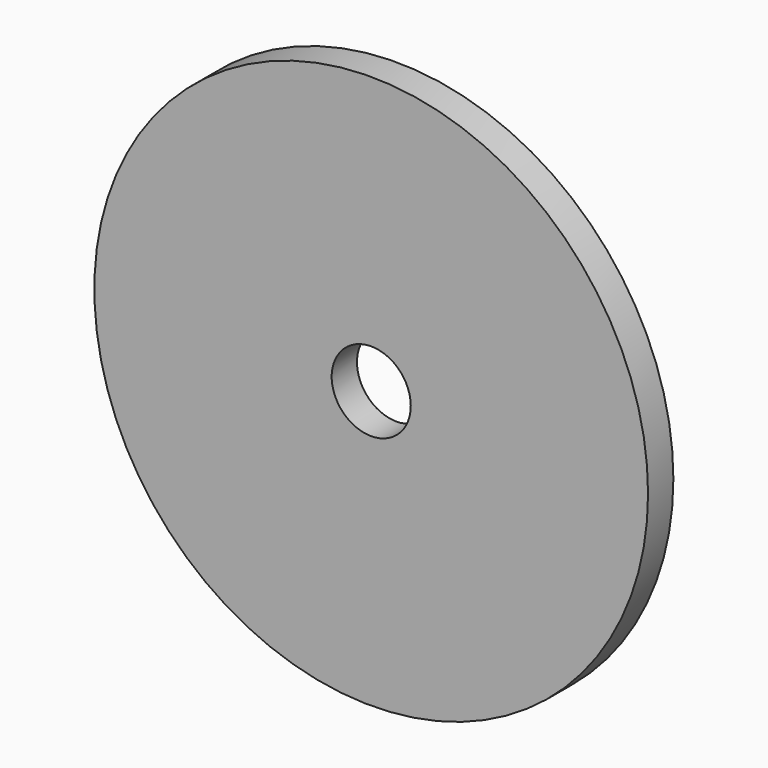
from build123d import *

# Parameters (mm, degrees)
F0_R     = 17.5
F1_DEPTH = 2.00000108
F2_R     = 2.5
F3_DEPTH = 6
F6_DEPTH = 8.00100108


# Not quite as in the source:
# - a feature of the source that left no trace in its solid (it failed there, or was rolled back) is left out


with BuildPart() as f1:
    # F0 (on Front) → F1 (new body)
    with BuildSketch(Plane.XZ):
        with Locations((-15.6701616943, 19.357258454)):
            Circle(F0_R)
    extrude(amount=F1_DEPTH)

    # F2 (on face) → F3 (join)
    with BuildSketch(Plane.XZ.offset(2.00000108)):
        with Locations((-15.6701616943, 19.357258454)):
            Circle(F2_R)
    extrude(amount=F3_DEPTH)

    # F6 (cut, through all): a face of the model
    f6_faces = [f1.faces().sort_by_distance(p)[0] for p in [
        (-15.6701616943, -8.00000108, 19.357258454),
    ]]
    extrude(f6_faces, amount=-F6_DEPTH, mode=Mode.SUBTRACT)


solid = f1.part
